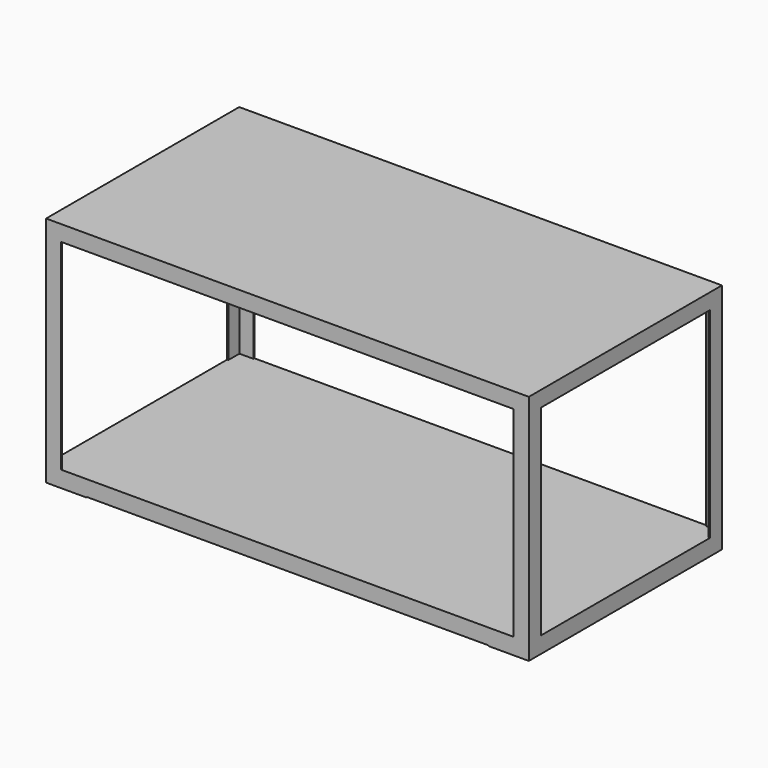
from build123d import *

# Parameters (mm, degrees)
F0_W      = 1219.2
F0_H      = 609.6
F1_DEPTH  = 1.51892
F2_W      = 1219.2
F2_H      = 609.6
F2_W_2    = 1216.16216
F2_H_2    = 606.56216
F3_DEPTH  = 38.1
F5_DEPTH  = 584.2
F7_W      = 1219.2
F7_H      = 609.6
F8_DEPTH  = 1.51892
F9_W      = 1219.2
F9_H      = 609.6
F9_W_2    = 1213.12432
F9_H_2    = 603.52432
F10_DEPTH = 38.1
F11_W     = 101.6
F11_H     = 609.6
F12_DEPTH = 1.51892
F13_R     = 1.5875
F14_DEPTH = 1.651


# Not quite as in the source:
# - a pattern or mirror of a feature is missing from the dataset's text; its kind, count and spacing are read off the source's solid


with BuildPart() as f1:
    # F0 (on Top) → F1 (new body)
    with BuildSketch(Plane.XY):
        Rectangle(F0_W, F0_H)
    extrude(amount=-F1_DEPTH)

    # F2 (on face) → F3 (join)
    with BuildSketch(Plane(origin=(0, 0, -1.51892), x_dir=(1, 0, 0), z_dir=(0, 0, -1))):
        Rectangle(F2_W, F2_H)
        Rectangle(F2_W_2, F2_H_2, mode=Mode.SUBTRACT)
    extrude(amount=F3_DEPTH)

    # F4 (on face) → F5 (join)
    with BuildSketch(Plane(origin=(0, 0, -1.51892), x_dir=(1, 0, 0), z_dir=(0, 0, -1))):
        Polygon((-571.5, 301.76216), (-571.5, 304.8), (-609.6, 304.8), (-609.6, 266.7), (-606.56216, 266.7), (-606.56216, 301.76216), align=None)
        Polygon((571.5, 304.8), (571.5, 301.76216), (606.56216, 301.76216), (606.56216, 266.7), (609.6, 266.7), (609.6, 304.8), align=None)
    f5 = extrude(amount=F5_DEPTH)

    # F5_copies: F5 across plane
    add(f5.mirror(Plane.ZX))

    # F7 (on offset) → F8 (join)
    with BuildSketch(Plane.XY.offset(-546.1)):
        Rectangle(F7_W, F7_H)
    extrude(amount=-F8_DEPTH)

    # F9 (on face) → F10 (join)
    with BuildSketch(Plane(origin=(0, 0, -547.61892), x_dir=(1, 0, 0), z_dir=(0, 0, -1))):
        Rectangle(F9_W, F9_H)
        Rectangle(F9_W_2, F9_H_2, mode=Mode.SUBTRACT)
    extrude(amount=F10_DEPTH)

    # F11 (on face) → F12 (join)
    with BuildSketch(Plane(origin=(0, 0, -585.71892), x_dir=(1, 0, 0), z_dir=(0, 0, -1))):
        with Locations((-558.8, 0)):
            Rectangle(F11_W, F11_H)
    f12 = extrude(amount=F12_DEPTH)

    # F12_copies: F12 across plane
    add(f12.mirror(Plane(origin=(0, 0, 0), x_dir=(0, 0, 1), z_dir=(1, 0, 0))))

    # F13 (on face) → F14 (cut)
    with BuildSketch(Plane(origin=(0, 0, -587.23784), x_dir=(1, 0, 0), z_dir=(0, 0, -1))):
        with Locations((-584.2, 285.75)):
            Circle(F13_R)
    f14 = extrude(amount=-F14_DEPTH, mode=Mode.SUBTRACT)

    # F14_copies: F14 across plane
    add(f14.mirror(Plane(origin=(0, 0, 0), x_dir=(0, 0, 1), z_dir=(1, 0, 0))), mode=Mode.SUBTRACT)

    # F14_copies1: F14 across plane
    add(f14.mirror(Plane.ZX), mode=Mode.SUBTRACT)

    # F14_copies2: F14 across plane
    add(f14.mirror(Plane(origin=(0, 0, 0), x_dir=(-0.4393852473, 0.8982987278, 0), z_dir=(0.8982987278, 0.4393852473, 0))), mode=Mode.SUBTRACT)


solid = f1.part
